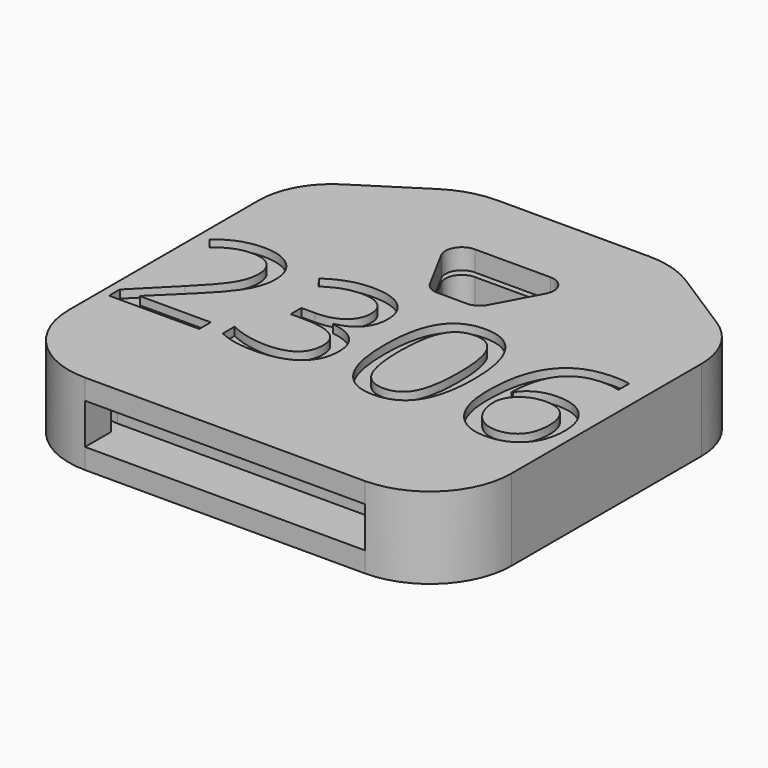
from build123d import *

# Parameters (mm, degrees)
F1_DEPTH       = 1
F2_R           = 3
F3_R           = 2
F4_R           = 2.5
F6_DEPTH       = 25
F7_R           = 1
F8_R           = 1
F10_DEPTH      = 3.5
F10_DEPTH_BACK = 1.5
F12_START      = 0.25
F12_DEPTH      = 1.25
F13_START      = 2.5
F13_DEPTH      = 1.25
F14_TEXT_SIZE  = 11.8108419839
F15_DEPTH      = 0.5


# Not quite as in the source:
# - Text() gives the source's letters only with a copy of the font that has no kerning and outlines rounded to 1/6400 em; it was checked with that copy


with BuildPart() as f1:
    # F0 (on Top) → F1 (new body, symmetric)
    with BuildSketch(Plane.XY):
        Polygon((-11.1, -10.875), (11.1, -10.875), (11.1, 7.315), (5.54, 10.875), (-5.54, 10.875), (-11.1, 7.315), align=None)
    extrude(amount=F1_DEPTH, both=True)

    # F2
    f2_edges = [f1.edges().sort_by_distance(p)[0] for p in [
        (-5.54, 10.875, 0),
        (5.54, 10.875, 0),
    ]]
    fillet(f2_edges, radius=F2_R)

    # F3
    f3_edges = [f1.edges().sort_by_distance(p)[0] for p in [
        (-11.1, 7.315, 0),
        (11.1, 7.315, 0),
    ]]
    fillet(f3_edges, radius=F3_R)

    # F4
    f4_edges = [f1.edges().sort_by_distance(p)[0] for p in [
        (-11.1, -10.875, 0),
        (11.1, -10.875, 0),
    ]]
    fillet(f4_edges, radius=F4_R)

    # F5 (on face) → F6 (cut)
    with BuildSketch(Plane.XY.offset(1)):
        Polygon((4, 8.725), (-4, 8.725), (-1.5, 4.075), (1.5, 4.075), align=None)
    extrude(amount=-F6_DEPTH, mode=Mode.SUBTRACT)

    # F7
    f7_edges = [f1.edges().sort_by_distance(p)[0] for p in [
        (-4, 8.725, 0),
        (4, 8.725, 0),
    ]]
    fillet(f7_edges, radius=F7_R)

    # F8
    f8_edges = [f1.edges().sort_by_distance(p)[0] for p in [
        (-1.5, 4.075, 0),
        (1.5, 4.075, 0),
    ]]
    fillet(f8_edges, radius=F8_R)


with BuildPart() as f10:
    # F9 (on face) → F10 (new body, two sides)
    with BuildSketch(Plane.XY.offset(1)) as f10_sk:
        with BuildLine():
            Line((-7.627600179, 12.5068874234), (-11.5265152558, 10.0104597843))
            ThreePointArc((-11.5265152558, 10.0104597843), (-13.0477410408, 8.3806736807), (-13.6, 6.2207337106))
            Line((-13.6, 6.2207337106), (-13.6, -8.375))
            ThreePointArc((-13.6, -8.375), (-12.1355339059, -11.9105339059), (-8.6, -13.375))
            Line((-8.6, -13.375), (-8.6, -11.375))
            ThreePointArc((-8.6, -11.375), (-10.7213203436, -10.4963203436), (-11.6, -8.375))
            Line((-11.6, -8.375), (-11.6, 6.2207337106))
            ThreePointArc((-11.6, 6.2207337106), (-11.2931894671, 7.4207003607), (-10.448064031, 8.3261370849))
            Line((-10.448064031, 8.3261370849), (-6.5491489542, 10.822564724))
            ThreePointArc((-6.5491489542, 10.822564724), (-5.6450997357, 11.2340531801), (-4.6618593108, 11.375))
            Line((-4.6618593108, 11.375), (4.6618593108, 11.375))
            ThreePointArc((4.6618593108, 11.375), (5.6450997357, 11.2340531801), (6.5491489542, 10.822564724))
            Line((6.5491489542, 10.822564724), (10.448064031, 8.3261370849))
            ThreePointArc((10.448064031, 8.3261370849), (11.2931894671, 7.4207003607), (11.6, 6.2207337106))
            Line((11.6, 6.2207337106), (11.6, -8.375))
            ThreePointArc((11.6, -8.375), (10.7213203436, -10.4963203436), (8.6, -11.375))
            Line((8.6, -11.375), (8.6, -13.375))
            ThreePointArc((8.6, -13.375), (12.1355339059, -11.9105339059), (13.6, -8.375))
            Line((13.6, -8.375), (13.6, 6.2207337106))
            ThreePointArc((13.6, 6.2207337106), (13.0477410408, 8.3806736807), (11.5265152558, 10.0104597843))
            Line((11.5265152558, 10.0104597843), (7.627600179, 12.5068874234))
            ThreePointArc((7.627600179, 12.5068874234), (6.206951407, 13.1535121402), (4.6618593108, 13.375))
            Line((4.6618593108, 13.375), (-4.6618593108, 13.375))
            ThreePointArc((-4.6618593108, 13.375), (-6.206951407, 13.1535121402), (-7.627600179, 12.5068874234))
        make_face()
    extrude(amount=-F10_DEPTH)
    extrude(f10_sk.sketch, amount=F10_DEPTH_BACK)

    # F11 (on face) → F12 (join)
    with BuildSketch(Plane.XY.offset(1).offset(F12_START)):
        with BuildLine():
            Line((-13.6, 6.2207337106), (-13.6, -8.375))
            ThreePointArc((-13.6, -8.375), (-12.1355339059, -11.9105339059), (-8.6, -13.375))
            Line((-8.6, -13.375), (8.6, -13.375))
            ThreePointArc((8.6, -13.375), (12.1355339059, -11.9105339059), (13.6, -8.375))
            Line((13.6, -8.375), (13.6, 6.2207337106))
            ThreePointArc((13.6, 6.2207337106), (13.0477410408, 8.3806736807), (11.5265152558, 10.0104597843))
            Line((11.5265152558, 10.0104597843), (7.627600179, 12.5068874234))
            ThreePointArc((7.627600179, 12.5068874234), (6.206951407, 13.1535121402), (4.6618593108, 13.375))
            Line((4.6618593108, 13.375), (-4.6618593108, 13.375))
            ThreePointArc((-4.6618593108, 13.375), (-6.206951407, 13.1535121402), (-7.627600179, 12.5068874234))
            Line((-7.627600179, 12.5068874234), (-11.5265152558, 10.0104597843))
            ThreePointArc((-11.5265152558, 10.0104597843), (-13.0477410408, 8.3806736807), (-13.6, 6.2207337106))
        make_face()
        with BuildLine():
            Line((11.1, 6.2207337106), (11.1, -8.375))
            ThreePointArc((11.1, -8.375), (10.367766953, -10.142766953), (8.6, -10.875))
            Line((8.6, -10.875), (-8.6, -10.875))
            ThreePointArc((-8.6, -10.875), (-10.367766953, -10.142766953), (-11.1, -8.375))
            Line((-11.1, -8.375), (-11.1, 6.2207337106))
            ThreePointArc((-11.1, 6.2207337106), (-10.8545515737, 7.1807070307), (-10.1784512248, 7.90505641))
            Line((-10.1784512248, 7.90505641), (-6.279536148, 10.4014840491))
            ThreePointArc((-6.279536148, 10.4014840491), (-5.5046368178, 10.7541884401), (-4.6618593108, 10.875))
            Line((-4.6618593108, 10.875), (4.6618593108, 10.875))
            ThreePointArc((4.6618593108, 10.875), (5.5046368178, 10.7541884401), (6.279536148, 10.4014840491))
            Line((6.279536148, 10.4014840491), (10.1784512248, 7.90505641))
            ThreePointArc((10.1784512248, 7.90505641), (10.8545515737, 7.1807070307), (11.1, 6.2207337106))
        make_face(mode=Mode.SUBTRACT)
        with BuildLine():
            ThreePointArc((8.6, -10.875), (10.367766953, -10.142766953), (11.1, -8.375))
            Line((11.1, -8.375), (11.1, 6.2207337106))
            ThreePointArc((11.1, 6.2207337106), (10.8545515737, 7.1807070307), (10.1784512248, 7.90505641))
            Line((10.1784512248, 7.90505641), (6.279536148, 10.4014840491))
            ThreePointArc((6.279536148, 10.4014840491), (5.5046368178, 10.7541884401), (4.6618593108, 10.875))
            Line((4.6618593108, 10.875), (-4.6618593108, 10.875))
            ThreePointArc((-4.6618593108, 10.875), (-5.5046368178, 10.7541884401), (-6.279536148, 10.4014840491))
            Line((-6.279536148, 10.4014840491), (-10.1784512248, 7.90505641))
            ThreePointArc((-10.1784512248, 7.90505641), (-10.8545515737, 7.1807070307), (-11.1, 6.2207337106))
            Line((-11.1, 6.2207337106), (-11.1, -8.375))
            ThreePointArc((-11.1, -8.375), (-10.367766953, -10.142766953), (-8.6, -10.875))
            Line((-8.6, -10.875), (8.6, -10.875))
        make_face()
        with BuildLine():
            ThreePointArc((2.3270018799, 8.725), (3.1853534859, 8.2380619071), (3.2077769037, 7.251465041))
            Line((3.2077769037, 7.251465041), (1.7830457209, 4.601465041))
            ThreePointArc((1.7830457209, 4.601465041), (1.4153326042, 4.216648394), (0.9022706971, 4.075))
            Line((0.9022706971, 4.075), (-0.9022706971, 4.075))
            ThreePointArc((-0.9022706971, 4.075), (-1.4153326042, 4.216648394), (-1.7830457209, 4.601465041))
            Line((-1.7830457209, 4.601465041), (-3.2077769037, 7.251465041))
            ThreePointArc((-3.2077769037, 7.251465041), (-3.1853534859, 8.2380619071), (-2.3270018799, 8.725))
            Line((-2.3270018799, 8.725), (2.3270018799, 8.725))
        make_face(mode=Mode.SUBTRACT)
    extrude(amount=F12_DEPTH)

    # F12_face (on face) → F13 (join)
    with BuildSketch(Plane(origin=(0, -1.5240715806, 1.25), x_dir=(1, 0, 0), z_dir=(0, 0, -1)).offset(F13_START)):
        with BuildLine():
            Line((-8.6, 11.8509284194), (-8.6, 9.8509284194))
            ThreePointArc((-8.6, 9.8509284194), (-10.7213203436, 8.9722487629), (-11.6, 6.8509284194))
            Line((-11.6, 6.8509284194), (-11.6, -7.7448052913))
            ThreePointArc((-11.6, -7.7448052913), (-11.2931894671, -8.9447719413), (-10.448064031, -9.8502086655))
            Line((-10.448064031, -9.8502086655), (-6.5491489542, -12.3466363046))
            ThreePointArc((-6.5491489542, -12.3466363046), (-5.6450997357, -12.7581247608), (-4.6618593108, -12.8990715806))
            Line((-4.6618593108, -12.8990715806), (4.6618593108, -12.8990715806))
            ThreePointArc((4.6618593108, -12.8990715806), (5.6450997357, -12.7581247608), (6.5491489542, -12.3466363046))
            Line((6.5491489542, -12.3466363046), (10.448064031, -9.8502086655))
            ThreePointArc((10.448064031, -9.8502086655), (11.2931894671, -8.9447719413), (11.6, -7.7448052913))
            Line((11.6, -7.7448052913), (11.6, 6.8509284194))
            ThreePointArc((11.6, 6.8509284194), (10.7213203436, 8.9722487629), (8.6, 9.8509284194))
            Line((8.6, 9.8509284194), (8.6, 11.8509284194))
            Line((8.6, 11.8509284194), (-8.6, 11.8509284194))
        make_face()
        with BuildLine():
            Line((1.7830457209, -6.1255366216), (3.2077769037, -8.7755366216))
            ThreePointArc((3.2077769037, -8.7755366216), (3.1853534859, -9.7621334877), (2.3270018799, -10.2490715806))
            Line((2.3270018799, -10.2490715806), (-2.3270018799, -10.2490715806))
            ThreePointArc((-2.3270018799, -10.2490715806), (-3.1853534859, -9.7621334877), (-3.2077769037, -8.7755366216))
            Line((-3.2077769037, -8.7755366216), (-1.7830457209, -6.1255366216))
            ThreePointArc((-1.7830457209, -6.1255366216), (-1.4153326042, -5.7407199746), (-0.9022706971, -5.5990715806))
            Line((-0.9022706971, -5.5990715806), (0.9022706971, -5.5990715806))
            ThreePointArc((0.9022706971, -5.5990715806), (1.4153326042, -5.7407199746), (1.7830457209, -6.1255366216))
        make_face(mode=Mode.SUBTRACT)
    extrude(amount=F13_DEPTH)

    # F14 (on face) → F15 (cut)
    with BuildSketch(Plane.XY.offset(2.5)):
        with Locations((-13.6, -6.0038062284)):
            Text('2306', F14_TEXT_SIZE, font='Open Sans', text_align=(TextAlign.LEFT, TextAlign.BOTTOM))
    extrude(amount=-F15_DEPTH, mode=Mode.SUBTRACT)


solid = Compound([f1.part, f10.part])
